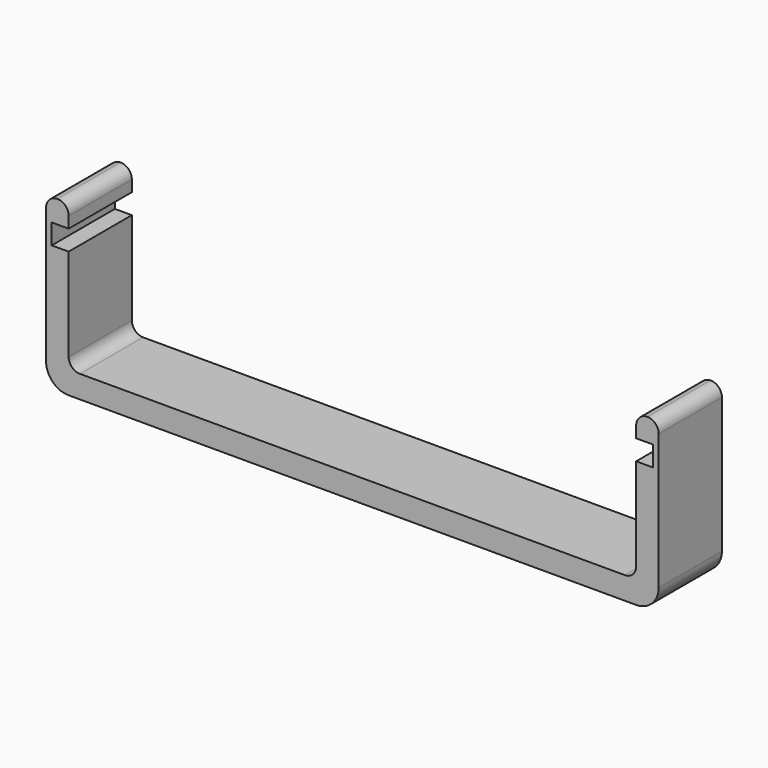
from build123d import *

# Parameters (mm, degrees)
F1_DEPTH = 7
F2_R     = 2
F3_R     = 1
F4_R     = 0.99999


# Not quite as in the source:
# - a fillet or chamfer is up to 0.001 mm smaller than in the source, because OpenCascade refuses the exact size


with BuildPart() as f1:
    # F0 (on Front) → F1 (new body)
    with BuildSketch(Plane.XZ):
        Polygon((-21.5481998797, -13.2900460566), (-23.5481998797, -13.2900460566), (-23.5481998797, -28.2900460566), (30.7518001203, -28.2900460566), (30.7518001203, -13.2900460566), (28.7518001203, -13.2900460566), (28.7518001203, -15.2900460566), (30.2518001203, -15.2900460566), (30.2518001203, -17.0800460566), (28.7518001203, -17.0800460566), (28.7518001203, -26.2900460566), (-21.5481998797, -26.2900460566), (-21.5481998797, -17.0800460566), (-23.0481998797, -17.0800460566), (-23.0481998797, -15.2900460566), (-21.5481998797, -15.2900460566), align=None)
    extrude(amount=F1_DEPTH)

    # F2
    f2_edges = [f1.edges().sort_by_distance(p)[0] for p in [
        (-23.5482, -3.5, -28.290046),
        (30.7518, -3.5, -28.290046),
    ]]
    fillet(f2_edges, radius=F2_R)

    # F3
    f3_edges = [f1.edges().sort_by_distance(p)[0] for p in [
        (-21.5482, -3.5, -26.290046),
        (28.7518, -3.5, -26.290046),
    ]]
    fillet(f3_edges, radius=F3_R)

    # F4 (radius 1 in the source; OpenCascade refuses exactly that, so slightly less here)
    f4_edges = [f1.edges().sort_by_distance(p)[0] for p in [
        (-23.5482, -3.5, -13.290046),
        (30.7518, -3.5, -13.290046),
        (-21.5482, -3.5, -13.290046),
        (28.7518, -3.5, -13.290046),
    ]]
    fillet(f4_edges, radius=F4_R)


solid = f1.part
